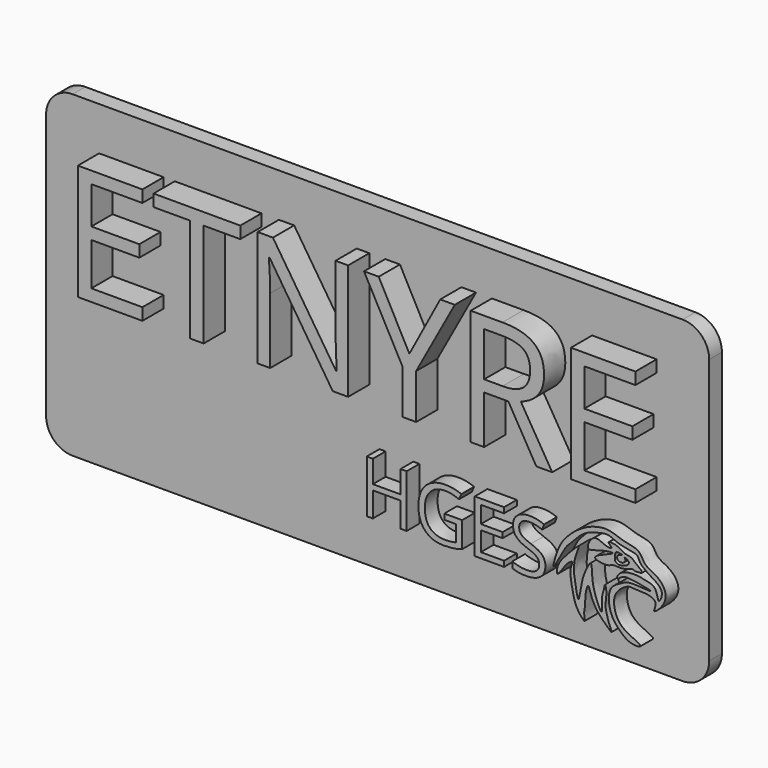
from build123d import *

# Parameters (mm, degrees)
F0_W          = 125
F0_H          = 60
F1_DEPTH      = 3
F2_TEXT_SIZE  = 13.8888888889
F3_DEPTH      = 3
F5_DEPTH      = 3
F7_DEPTH      = 3
F9_DEPTH      = 3
F11_DEPTH     = 3
F12_R         = 5
F13_TEXT_SIZE = 30.5555555556
F14_DEPTH     = 5


# Not quite as in the source:
# - Text() gives the source's letters only with a copy of the font that has no kerning and outlines rounded to 1/6400 em; it was checked with that copy


with BuildPart() as f1:
    # F0 (on Front) → F1 (new body)
    with BuildSketch(Plane.XZ):
        with Locations((-12.5, 15)):
            Rectangle(F0_W, F0_H)
    extrude(amount=-F1_DEPTH)

    # F2 (on face) → F3 (join)
    with BuildSketch(Plane.XZ):
        with Locations((-13.5143961917, -5)):
            Text('HGES', F2_TEXT_SIZE, font='Open Sans', text_align=(TextAlign.LEFT, TextAlign.BOTTOM))
    extrude(amount=F3_DEPTH)

    # F4 (on face) → F5 (join)
    with BuildSketch(Plane.XZ):
        with BuildLine():
            add(Edge.make_bspline(
                [(23.8162260503, -1.6755688703), (24.1360523759, -0.6575972668), (25.7231504486, 1.0727845273), (28.259531834, 3.7111779221), (27.1372368273, 1.2604371849), (26.7768007825, -1.036938774), (27.1606238788, -3.6081198491), (27.770407849, -6.6093505764), (28.092379912, -4.0735390436), (28.5871570991, -1.7405900159), (29.2988188955, -0.2041079215), (30.280883956, 1.6432138625), (30.3158513257, -1.1386430588), (30.4800656541, -2.4351573269), (30.9185217156, -4.2927695373), (32.4221933191, -7.6159083326), (31.9769895023, -3.9842138731), (32.6213106466, -2.6714026177), (32.7392625928, -1.304503102), (33.185167646, -3.1578190015), (32.6928365856, -4.9828869134), (33.0979990662, -6.6394148726), (33.4656398253, -7.9550270077), (34.4656796969, -9.7961867654), (32.4405554375, -7.9280782136), (31.023194078, -6.3699439418), (30.0941740502, -4.4414986908), (29.5899324739, -2.2918364015), (28.9283722618, -4.7963568366), (29.1226714439, -6.5202052986), (28.6670210741, -7.6919969387), (29.2661867588, -9.7109781903), (27.4816615018, -7.6089620441), (26.8676407752, -5.908760187), (26.3835842843, -3.4466571293), (26.0854993517, -1.1831039262), (26.9188816043, 0.3845016686), (25.2759591602, -0.6322619449), (23.6310977208, -3.7273449289), (23.6366462116, -2.2471515126), (23.8162260503, -1.6755688703)],
                knots=[0, 0, 0, 0, 0.0375977184, 0.0676221393, 0.0913725898, 0.1224880155, 0.1559755773, 0.1829182392, 0.2064966677, 0.2383034913, 0.2652905965, 0.286077174, 0.3126631227, 0.3366740597, 0.3654218498, 0.3941588146, 0.4229386213, 0.4497376699, 0.4659396087, 0.4872886573, 0.5155441792, 0.540289367, 0.5648655583, 0.5859221944, 0.6115391224, 0.6419583046, 0.6716694211, 0.6936890587, 0.7188737585, 0.7459450991, 0.7686011347, 0.7897388087, 0.8152954013, 0.8435507528, 0.8742544016, 0.904647068, 0.924517085, 0.9469653705, 0.9788891918, 1, 1, 1, 1], degree=3))
        make_face()
    extrude(amount=F5_DEPTH)

    # F6 (on face) → F7 (join)
    with BuildSketch(Plane.XZ):
        with BuildLine():
            add(Edge.make_bspline(
                [(23.1035146862, -1.8576275324), (22.9076155793, -1.8805807886), (23.8061852944, 1.5755198103), (25.5415339997, 4.0308552501), (28.6935646366, 6.6776212756), (33.0957147396, 8.0435649543), (36.0951891339, 6.4854228162), (39.4194735036, 6.2527826543), (40.0116112479, 3.9809870698), (42.051772758, 3.2157630609), (44.0848446229, 1.613501515), (44.5298171283, -1.1426105938), (41.3821640982, -4.0242489465), (42.7860863991, -1.4679303199), (40.8813468714, -0.6236041636), (38.4854161464, -0.7697624533), (37.0557943567, -0.3639456275), (34.7981311939, -2.1324024156), (34.385286482, -3.8219492246), (34.5769727021, -5.4236481221), (35.5585095291, -8.1436941912), (40.7739741984, -9.8302768713), (37.453744273, -10.1902093229), (35.3273679931, -8.33377401), (33.5464110842, -6.1999287598), (33.1896454935, -1.7725406386), (35.7815499219, -0.6386075587), (36.9608769141, 0.2174728525), (39.5274379855, 0.0015555289), (42.8365096843, -0.1498105113), (37.2465056933, 0.900751182), (36.0267248552, 0.7338339908), (34.7130579931, -0.4407120158), (35.4701813769, 1.5364223072), (38.5411446134, 1.8921586566), (40.4524039338, 1.4450575516), (42.547620883, 1.0323681983), (42.75394837, -1.965298157), (43.7360768128, 0.1828264616), (43.0486102966, 1.5591274214), (40.6881602619, 2.777881146), (39.1670239586, 4.0914491062), (39.0582852167, 5.2059992782), (37.2950805743, 5.503244901), (34.9910476681, 5.9015013202), (33.4018159046, 6.9127526704), (31.3075343055, 6.4281070829), (28.6613933367, 5.7164618234), (26.3467268904, 3.0226703455), (25.2048071023, 2.1672741396), (23.3353482259, -1.8304638833), (23.1035146862, -1.8576275324)],
                knots=[0, 0, 0, 0, 0.0230611886, 0.0484406729, 0.0753723235, 0.1034043942, 0.1280743215, 0.1513055801, 0.1700134404, 0.1893491139, 0.2104800466, 0.2325599513, 0.2543868591, 0.2701160072, 0.2873884012, 0.3084917496, 0.3245556412, 0.3462383739, 0.3636647503, 0.3802126518, 0.4034713855, 0.4295698657, 0.4465446048, 0.4695429203, 0.4922780091, 0.5187788585, 0.5397245631, 0.5556336561, 0.578352069, 0.5952851944, 0.622067898, 0.6396428672, 0.6528739247, 0.6672486415, 0.6905842562, 0.7101284458, 0.72884945, 0.7470227817, 0.7621912092, 0.7786495561, 0.8006754003, 0.819515811, 0.8321756495, 0.849077272, 0.8700930027, 0.8880425929, 0.9070414882, 0.9295892633, 0.9538408637, 0.97270862, 1, 1, 1, 1], degree=3))
        make_face()
    extrude(amount=F7_DEPTH)

    # F8 (on face) → F9 (join)
    with BuildSketch(Plane.XZ):
        with BuildLine():
            add(Edge.make_bspline(
                [(39.7617183626, 2.5405762717), (39.7364197953, 2.3977069692), (39.0321041033, 2.3596339861), (38.3877229562, 2.2868874479), (37.8347511166, 2.6772922774), (36.1020140363, 1.7411198447), (34.2947878692, 2.2268391215), (33.3321954607, 1.3514298943), (28.9202529375, 2.0959184578), (35.9759198891, 4.2673423444), (31.9061350681, 3.8553336819), (28.7013300108, 2.3829379257), (30.5716644397, 6.2412741838), (32.6902125618, 4.6153680495), (34.5144298803, 4.6194029181), (32.7450370489, 5.773738766), (35.3263432171, 5.5458084483), (36.2517490934, 4.5284490956), (37.6795016835, 4.5164543012), (38.4231443102, 3.7284249715), (39.8008145995, 2.761365538), (39.7617183626, 2.5405762717)],
                knots=[0, 0, 0, 0, 0.0349496175, 0.0703397301, 0.1015118955, 0.1584571747, 0.2136188522, 0.2641454437, 0.3266539254, 0.4076787913, 0.4681634469, 0.5363939097, 0.5999702347, 0.6650296031, 0.7076466606, 0.747033294, 0.8000707914, 0.8527299954, 0.898935591, 0.9459890945, 1, 1, 1, 1], degree=3))
        make_face()
    extrude(amount=F9_DEPTH)

    # F10 (on face) → F11 (cut)
    with BuildSketch(Plane.XZ.offset(3)):
        with BuildLine():
            add(Edge.make_bspline(
                [(36.0182896256, 4.1956356727), (36.0420621963, 4.2264392284), (35.6052656692, 4.3803031572), (34.7768729365, 4.4720303363), (34.6291512443, 3.7679465083), (34.4990427097, 2.2460913144), (36.631324823, 2.4393642296), (37.6644509235, 3.4581867722), (36.170223025, 4.1992649607), (36.8112631907, 3.4639398652), (36.0479951205, 2.754094666), (34.8972443643, 3.0334362348), (35.1099545676, 4.1938425291), (35.9853335696, 4.1529325201), (36.0182896256, 4.1956356727)],
                knots=[0, 0, 0, 0, 0.0563230207, 0.1368204352, 0.2082721444, 0.3065818284, 0.4277041696, 0.5203020239, 0.6069952546, 0.6673077931, 0.750758259, 0.8388761009, 0.9219190615, 1, 1, 1, 1], degree=3))
        make_face()
    extrude(amount=-F11_DEPTH, mode=Mode.SUBTRACT)

    # F12
    f12_edges = [f1.edges().sort_by_distance(p)[0] for p in [
        (-75, 1.5, 45),
        (50, 1.5, -15),
        (50, 1.5, 45),
        (-75, 1.5, -15),
    ]]
    fillet(f12_edges, radius=F12_R)

    # F13 (on face) → F14 (join)
    with BuildSketch(Plane.XZ):
        with Locations((-68, 15)):
            Text('ETNYRE', F13_TEXT_SIZE, font='Open Sans', text_align=(TextAlign.LEFT, TextAlign.BOTTOM))
    extrude(amount=F14_DEPTH)


solid = f1.part
